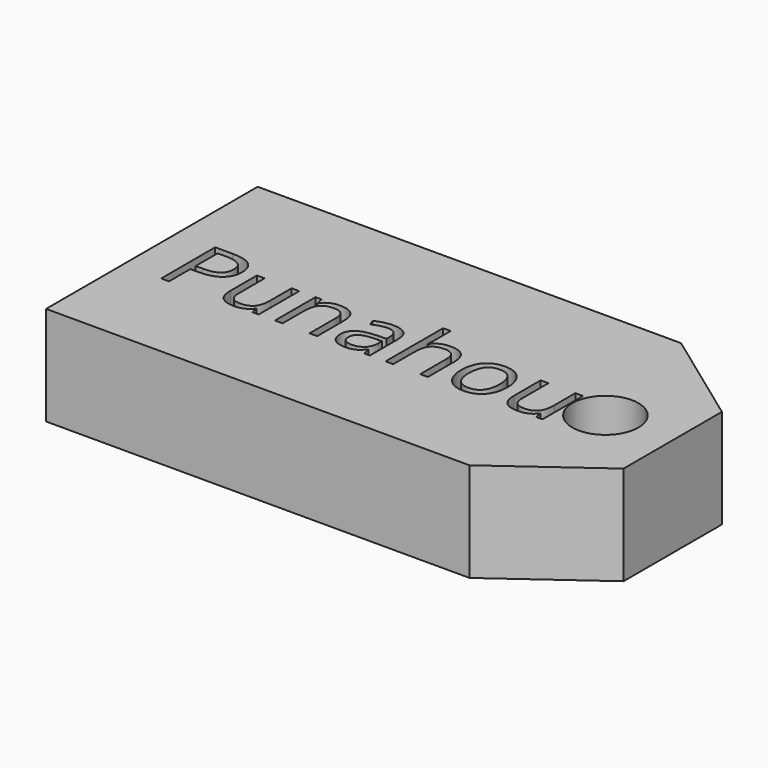
from build123d import *

# Parameters (mm, degrees)
F0_R         = 3.175
F1_DEPTH     = 9.525
F2_TEXT_SIZE = 9.0798733942
F3_DEPTH     = 25.4


# Not quite as in the source:
# - Text() gives the source's letters only with a copy of the font that has no kerning and outlines rounded to 1/6400 em; it was checked with that copy


with BuildPart() as f1:
    # F0 (on Top) → F1 (new body)
    with BuildSketch(Plane.XY):
        Polygon((-15.2667295207, -13.0267653942), (-15.2667295207, -25.7267653942), (-15.2667295207, -38.4267653942), (25.395551737, -38.4267653942), (34.7534483983, -31.6311512094), (34.7534483983, -25.7267653942), (34.7534483983, -19.822379579), (25.395551737, -13.0267653942), align=None)
        with Locations((28.286146, -25.7267653942)):
            Circle(F0_R, mode=Mode.SUBTRACT)
    extrude(amount=F1_DEPTH)

    # F2 (on face) → F3 (cut)
    with BuildSketch(Plane.XY.offset(9.525)):
        with Locations((-12.5034973728, -29.179076856)):
            Text('Punahou', F2_TEXT_SIZE, font='Open Sans', text_align=(TextAlign.LEFT, TextAlign.BOTTOM))
    extrude(amount=-F3_DEPTH, mode=Mode.SUBTRACT)


solid = f1.part
